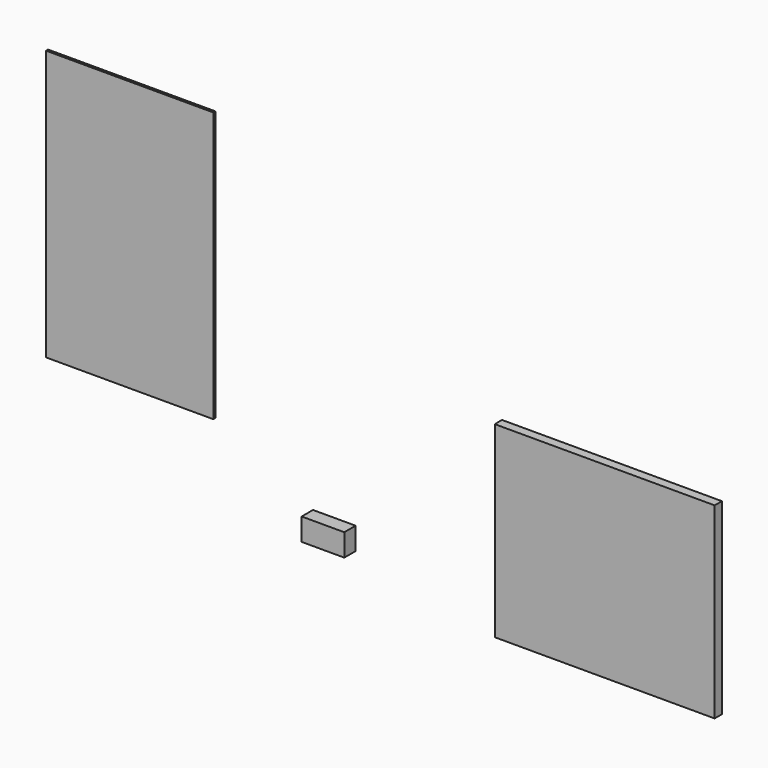
from build123d import *

# Parameters (mm, degrees)
F1_DEPTH = 0.635
F2_DEPTH = 3.556
F3_DEPTH = 2.286


with BuildPart() as f1:
    # F0 (on Front) → F1 (new body)
    with BuildSketch(Plane.XZ):
        Polygon((-29.3124206364, 39.8206487298), (-71.3453218341, 39.8206487298), (-71.3453218341, -28.0219372362), (-61.021450907, -28.0219372362), (-48.3009703457, -28.0219372362), (-29.3124206364, -28.0219372362), align=None)
    extrude(amount=F1_DEPTH)


with BuildPart() as f2:
    # F0 (on Front) → F2 (new body)
    with BuildSketch(Plane.XZ):
        Polygon((-4.7940909863, -40.3737090528), (-4.7940909863, -43.1860495352), (-4.7940909863, -45.9983900177), (5.9134630722, -45.9983900177), (5.9134630722, -40.3737090528), align=None)
    extrude(amount=F2_DEPTH)


with BuildPart() as f3:
    # F0 (on Front) → F3 (new body)
    with BuildSketch(Plane.XZ):
        Polygon((97.9521423578, -5.0171883777), (42.7046529949, -5.0171883777), (42.7046529949, -25.2566132694), (42.7046529949, -52.1529465914), (97.9521423578, -52.1529465914), align=None)
    extrude(amount=F3_DEPTH)


solid = Compound([f1.part, f2.part, f3.part])
